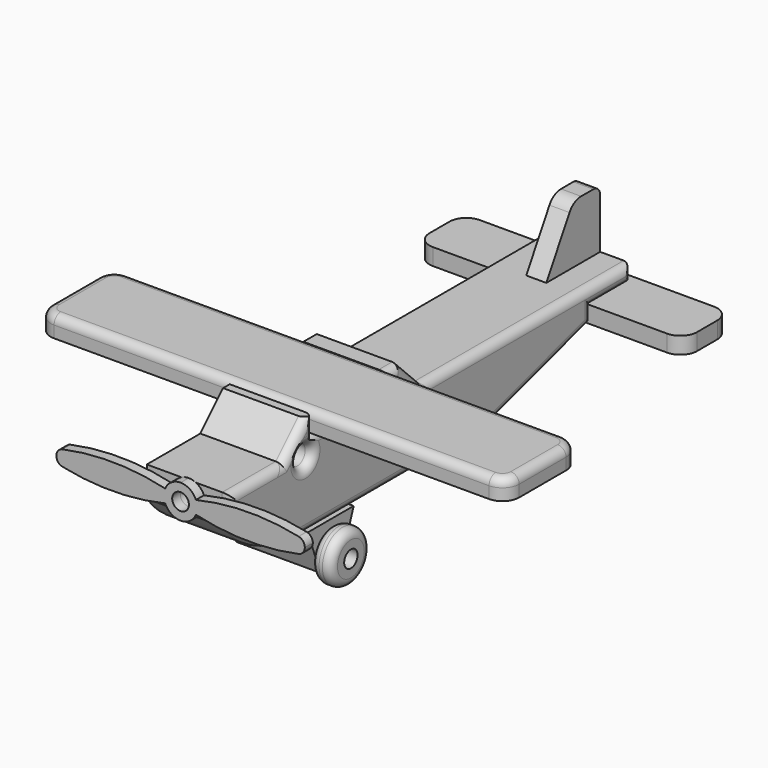
from build123d import *

# Parameters (mm, degrees)
F0_R           = 6
F1_DEPTH       = 25
F1_DEPTH_BACK  = 25
F2_W           = 55
F2_H           = 12
F3_DEPTH       = 140
F3_DEPTH_BACK  = 140
F4_R           = 10
F5_R           = 5
F6_W           = 35
F6_H           = 10
F7_DEPTH       = 80
F7_DEPTH_BACK  = 80
F8_R           = 10
F10_DEPTH      = 6
F10_DEPTH_BACK = 6
F11_R          = 10
F12_R          = 5
F13_R          = 5
F14_DEPTH      = 25
F14_DEPTH_BACK = 25
F15_R          = 15
F15_R_2        = 5
F16_DEPTH      = 12
F17_R          = 5
F18_R          = 5
F19_DEPTH      = 10
F20_R          = 5
F21_DEPTH      = 6
F22_R          = 4
F23_DEPTH      = 5
F24_R          = 4
F25_DEPTH      = 6
F26_T1_DEPTH   = 43.0048285071
F26_T3_DEPTH   = 162.520132507
F26_T5_DEPTH   = 117.2789705559
F26_T7_DEPTH   = 21.5024142536
F26_T9_DEPTH   = 42.5024142536
F26_T11_DEPTH  = 35.0048285071
F26_T13_DEPTH  = 35.0048285071
F26_T15_DEPTH  = 22.5024142536
F26_T17_DEPTH  = 55
F26_T20_ANGLE  = 66.2553378767
F26_T24_DEPTH  = 181.0048285071
F26_T29_DEPTH  = 49.0464590675
F26_T34_DEPTH  = 49.0464590675
F26_T39_DEPTH  = 65.0048285071
F26_T47_DEPTH  = 34.0048285071
F26_T52_DEPTH  = 42.5024142536
F26_T59_DEPTH  = 168.5024142536
F26_T63_DEPTH  = 49.0464590675
F26_T70_DEPTH  = 22.5024142536
F26_T74_DEPTH  = 67.5024142536
F26_T81_DEPTH  = 67.5024142536
F26_S83_R      = 6
F26_T84_DEPTH  = 35
F26_T87_DEPTH  = 22.5024142536
F26_S89_R      = 6
F26_T90_DEPTH  = 13
F26_T96_DEPTH  = 52.5024142536
F26_S98_R      = 6
F26_T99_DEPTH  = 28
F26_T102_DEPTH = 49.0464590675


# Not quite as in the source:
# - a fillet or chamfer that OpenCascade refuses, or shapes differently, is made with other operations: its cross-section is extruded or revolved along the edge and cut away or added


with BuildPart() as f1:
    # F0 (on Right) → F1 (new body, two sides)
    with BuildSketch(Plane.YZ) as f1_sk:
        with BuildLine():
            Line((-150, 18), (-150, 0))
            ThreePointArc((-150, 0), (-128.6521561512, -18.3853912602), (-101.266028276, -25))
            Line((-101.266028276, -25), (40, -25))
            Line((40, -25), (120, -1))
            Line((120, -1), (120, 8))
            Line((120, 8), (150, 8))
            Line((150, 8), (150, 18))
            Line((150, 18), (-6, 18))
            Line((-6, 18), (-23, 35))
            Line((-23, 35), (-33, 35))
            Line((-33, 35), (-33, 25))
            Line((-33, 25), (-88, 25))
            Line((-88, 25), (-88, 35))
            Line((-88, 35), (-93, 35))
            Line((-93, 35), (-110, 18))
            Line((-110, 18), (-150, 18))
        make_face()
        with Locations((-94, 15)):
            Circle(F0_R, mode=Mode.SUBTRACT)
    extrude(amount=F1_DEPTH)
    extrude(f1_sk.sketch, amount=-F1_DEPTH_BACK)

    # F18 (on face) → F19 (cut)
    with BuildSketch(Plane.XZ.offset(150)):
        with Locations((0, 9)):
            Circle(F18_R)
    extrude(amount=-F19_DEPTH, mode=Mode.SUBTRACT)

    # F24 (on face) → F25 (cut)
    with BuildSketch(Plane(origin=(0, 0, -25), x_dir=(1, 0, 0), z_dir=(0, 0, -1))):
        with Locations((-12, 75)):
            Circle(F24_R)
        with Locations((12, 75)):
            Circle(F24_R)
    extrude(amount=-F25_DEPTH, mode=Mode.SUBTRACT)

    # F26: fillet of radius 5 on 17 edges, made by hand

    # F26_s2 → F26_t1 (cut)
    with BuildSketch(Plane.XY.offset(-12.5024142536)):
        with BuildLine():
            ThreePointArc((19.9990343146, -150.0004), (23.5355339059, -148.5355339059), (25.0004, -144.9990343146))
            Line((25.0004, -144.9990343146), (25.5005365685, -144.9990343146))
            ThreePointArc((25.5005365685, -144.9990343146), (25.5001365685, -147.4995171573), (25.5001365685, -150))
            Line((25.5001365685, -150), (25, -150.5001365685))
            ThreePointArc((25, -150.5001365685), (22.4995171573, -150.5001365685), (19.9990343146, -150.5005365685))
            Line((19.9990343146, -150.5005365685), (19.9990343146, -150.0004))
        make_face()
    extrude(amount=F26_T1_DEPTH, mode=Mode.SUBTRACT)

    # F26_s4 → F26_t3 (cut)
    with BuildSketch(Plane.XZ.offset(-61.254104231)):
        with BuildLine():
            ThreePointArc((25.0004, -19.9990343146), (23.5355339059, -23.5355339059), (19.9990343146, -25.0004))
            Line((19.9990343146, -25.0004), (19.9990343146, -25.5005365685))
            ThreePointArc((19.9990343146, -25.5005365685), (22.4995171573, -25.5001365685), (25, -25.5001365685))
            Line((25, -25.5001365685), (25.5001365685, -25))
            ThreePointArc((25.5001365685, -25), (25.5001365685, -22.4995171573), (25.5005365685, -19.9990343146))
            Line((25.5005365685, -19.9990343146), (25.0004, -19.9990343146))
        make_face()
    extrude(amount=F26_T3_DEPTH, mode=Mode.SUBTRACT)

    # F26_s6 → F26_t5 (cut)
    with BuildSketch(Plane(origin=(0, 9.4587740601, 2.837632218), x_dir=(1, 0, 0), z_dir=(0, 0.9578262852, 0.2873478856))):
        with BuildLine():
            ThreePointArc((25.0004, 30.4386068678), (23.5355339059, 33.9751064591), (19.9990343146, 35.4399725532))
            Line((19.9990343146, 35.4399725532), (19.9990343146, 35.9401091217))
            ThreePointArc((19.9990343146, 35.9401091217), (22.4995171573, 35.9397091217), (25, 35.9397091217))
            Line((25, 35.9397091217), (25.5001365685, 35.4395725532))
            ThreePointArc((25.5001365685, 35.4395725532), (25.5001365685, 32.9390897105), (25.5005365685, 30.4386068678))
            Line((25.5005365685, 30.4386068678), (25.0004, 30.4386068678))
        make_face()
    extrude(amount=F26_T5_DEPTH, mode=Mode.SUBTRACT)

    # F26_s8 → F26_t7 (cut)
    with BuildSketch(Plane.XY.offset(-13.5024142536)):
        with BuildLine():
            ThreePointArc((25.0004, 114.9990343146), (23.5355339059, 118.5355339059), (19.9990343146, 120.0004))
            Line((19.9990343146, 120.0004), (19.9990343146, 120.5005365685))
            ThreePointArc((19.9990343146, 120.5005365685), (22.4995171573, 120.5001365685), (25, 120.5001365685))
            Line((25, 120.5001365685), (25.5001365685, 120))
            ThreePointArc((25.5001365685, 120), (25.5001365685, 117.4995171573), (25.5005365685, 114.9990343146))
            Line((25.5005365685, 114.9990343146), (25.0004, 114.9990343146))
        make_face()
    extrude(amount=F26_T7_DEPTH, mode=Mode.SUBTRACT)

    # F26_s10 → F26_t9 (cut)
    with BuildSketch(Plane.XZ.offset(-162.5024142536)):
        with BuildLine():
            ThreePointArc((25.0004, 13.0009656854), (23.5355339059, 9.4644660941), (19.9990343146, 7.9996))
            Line((19.9990343146, 7.9996), (19.9990343146, 7.4994634315))
            ThreePointArc((19.9990343146, 7.4994634315), (22.4995171573, 7.4998634315), (25, 7.4998634315))
            Line((25, 7.4998634315), (25.5001365685, 8))
            ThreePointArc((25.5001365685, 8), (25.5001365685, 10.5004828427), (25.5005365685, 13.0009656854))
            Line((25.5005365685, 13.0009656854), (25.0004, 13.0009656854))
        make_face()
    extrude(amount=F26_T9_DEPTH, mode=Mode.SUBTRACT)

    # F26_s12 → F26_t11 (cut)
    with BuildSketch(Plane.XY.offset(-4.5024142536)):
        with BuildLine():
            ThreePointArc((25.0004, 144.9990343146), (23.5355339059, 148.5355339059), (19.9990343146, 150.0004))
            Line((19.9990343146, 150.0004), (19.9990343146, 150.5005365685))
            ThreePointArc((19.9990343146, 150.5005365685), (22.4995171573, 150.5001365685), (25, 150.5001365685))
            Line((25, 150.5001365685), (25.5001365685, 150))
            ThreePointArc((25.5001365685, 150), (25.5001365685, 147.4995171573), (25.5005365685, 144.9990343146))
            Line((25.5005365685, 144.9990343146), (25.0004, 144.9990343146))
        make_face()
    extrude(amount=F26_T11_DEPTH, mode=Mode.SUBTRACT)

    # F26_s14 → F26_t13 (cut)
    with BuildSketch(Plane.XZ.offset(10.4975857464)):
        with BuildLine():
            ThreePointArc((25.0004, 29.9990343146), (23.5355339059, 33.5355339059), (19.9990343146, 35.0004))
            Line((19.9990343146, 35.0004), (19.9990343146, 35.5005365685))
            ThreePointArc((19.9990343146, 35.5005365685), (22.4995171573, 35.5001365685), (25, 35.5001365685))
            Line((25, 35.5001365685), (25.5001365685, 35))
            ThreePointArc((25.5001365685, 35), (25.5001365685, 32.4995171573), (25.5005365685, 29.9990343146))
            Line((25.5005365685, 29.9990343146), (25.0004, 29.9990343146))
        make_face()
    extrude(amount=F26_T13_DEPTH, mode=Mode.SUBTRACT)

    # F26_s16 → F26_t15 (cut)
    with BuildSketch(Plane.XY.offset(25)):
        with BuildLine():
            ThreePointArc((25.0004, -27.9990343146), (23.5355339059, -31.5355339059), (19.9990343146, -33.0004))
            Line((19.9990343146, -33.0004), (19.9990343146, -33.5005365685))
            ThreePointArc((19.9990343146, -33.5005365685), (22.4995171573, -33.5001365685), (25, -33.5001365685))
            Line((25, -33.5001365685), (25.5001365685, -33))
            ThreePointArc((25.5001365685, -33), (25.5001365685, -30.4995171573), (25.5005365685, -27.9990343146))
            Line((25.5005365685, -27.9990343146), (25.0004, -27.9990343146))
        make_face()
        with BuildLine():
            ThreePointArc((25.0004, -93.0009656854), (23.5355339059, -89.4644660941), (19.9990343146, -87.9996))
            Line((19.9990343146, -87.9996), (19.9990343146, -87.4994634315))
            ThreePointArc((19.9990343146, -87.4994634315), (22.4995171573, -87.4998634315), (25, -87.4998634315))
            Line((25, -87.4998634315), (25.5001365685, -88))
            ThreePointArc((25.5001365685, -88), (25.5001365685, -90.5004828427), (25.5005365685, -93.0009656854))
            Line((25.5005365685, -93.0009656854), (25.0004, -93.0009656854))
        make_face()
    extrude(amount=F26_T15_DEPTH, mode=Mode.SUBTRACT)

    # F26_s18 → F26_t17 (cut)
    with BuildSketch(Plane.XZ.offset(33)):
        with BuildLine():
            ThreePointArc((25.0004, 19.9990343146), (23.5355339059, 23.5355339059), (19.9990343146, 25.0004))
            Line((19.9990343146, 25.0004), (19.9990343146, 25.5005365685))
            ThreePointArc((19.9990343146, 25.5005365685), (22.4995171573, 25.5001365685), (25, 25.5001365685))
            Line((25, 25.5001365685), (25.5001365685, 25))
            ThreePointArc((25.5001365685, 25), (25.5001365685, 22.4995171573), (25.5005365685, 19.9990343146))
            Line((25.5005365685, 19.9990343146), (25.0004, 19.9990343146))
        make_face()
    extrude(amount=F26_T17_DEPTH, mode=Mode.SUBTRACT)

    # F26_s19 → F26_t20 (revolve, cut)
    with BuildSketch(Plane(origin=(0, -29.3190407601, 66.6494319351), x_dir=(1, 0, 0), z_dir=(0, -0.4026614145, 0.9153489964))):
        with BuildLine():
            ThreePointArc((25.0004, -133.5996421648), (23.5355339059, -137.1361417561), (19.9990343146, -138.6010078502))
            Line((19.9990343146, -138.6010078502), (19.9990343146, -139.1011444188))
            ThreePointArc((19.9990343146, -139.1011444188), (22.4995171573, -139.1007444188), (25, -139.1007444188))
            Line((25, -139.1007444188), (25.5001365685, -138.6006078502))
            ThreePointArc((25.5001365685, -138.6006078502), (25.5001365685, -136.1001250075), (25.5005365685, -133.5996421648))
            Line((25.5005365685, -133.5996421648), (25.0004, -133.5996421648))
        make_face()
    revolve(axis=Axis((25, -101.266028276, 35), (1, 0, 0)), revolution_arc=F26_T20_ANGLE, mode=Mode.SUBTRACT)


with BuildPart() as f3:
    # F2 (on Right) → F3 (new body, two sides)
    with BuildSketch(Plane.YZ) as f3_sk:
        with Locations((-60.5, 31)):
            Rectangle(F2_W, F2_H)
    extrude(amount=F3_DEPTH)
    extrude(f3_sk.sketch, amount=-F3_DEPTH_BACK)

    # F4
    f4_edges = [f3.edges().sort_by_distance(p)[0] for p in [
        (140, -88, 31),
        (140, -33, 31),
        (-140, -88, 31),
        (-140, -33, 31),
    ]]
    fillet(f4_edges, radius=F4_R)

    # F5
    f5_edges = [f3.edges().sort_by_distance(p)[0] for p in [
        (0, -33, 37),
        (137.071068, -35.928932, 37),
        (-137.071068, -35.928932, 37),
        (140, -60.5, 37),
        (-140, -60.5, 37),
        (137.071068, -85.071068, 37),
        (-137.071068, -85.071068, 37),
        (0, -88, 37),
    ]]
    fillet(f5_edges, radius=F5_R)


with BuildPart() as f7:
    # F6 (on Right) → F7 (new body, two sides)
    with BuildSketch(Plane.YZ) as f7_sk:
        with Locations((137.5, 3)):
            Rectangle(F6_W, F6_H)
    extrude(amount=F7_DEPTH)
    extrude(f7_sk.sketch, amount=-F7_DEPTH_BACK)

    # F8
    f8_edges = [f7.edges().sort_by_distance(p)[0] for p in [
        (80, 120, 3),
        (80, 155, 3),
        (-80, 155, 3),
        (-80, 120, 3),
    ]]
    fillet(f8_edges, radius=F8_R)


with BuildPart() as f10:
    # F9 (on Right) → F10 (new body, two sides)
    with BuildSketch(Plane.YZ) as f10_sk:
        Polygon((130, 53), (109.7927405784, 18), (150, 18), (150, 53), align=None)
    extrude(amount=F10_DEPTH)
    extrude(f10_sk.sketch, amount=-F10_DEPTH_BACK)

    # F11
    f11_edges = [f10.edges().sort_by_distance(p)[0] for p in [
        (0, 130, 53),
    ]]
    fillet(f11_edges, radius=F11_R)

    # F12
    f12_edges = [f10.edges().sort_by_distance(p)[0] for p in [
        (0, 150, 53),
    ]]
    fillet(f12_edges, radius=F12_R)


with BuildPart() as f14:
    # F13 (on Right) → F14 (new body, two sides)
    with BuildSketch(Plane.YZ) as f14_sk:
        Polygon((-67, -50), (-57.9007441433, -25), (-92.0992558567, -25), (-83, -50), align=None)
        with Locations((-75, -42)):
            Circle(F13_R, mode=Mode.SUBTRACT)
    extrude(amount=F14_DEPTH)
    extrude(f14_sk.sketch, amount=-F14_DEPTH_BACK)

    # F22 (on face) → F23 (cut)
    with BuildSketch(Plane.XY.offset(-25)):
        with Locations((-12, -75)):
            Circle(F22_R)
        with Locations((12, -75)):
            Circle(F22_R)
    extrude(amount=-F23_DEPTH, mode=Mode.SUBTRACT)


with BuildPart() as f16:
    # F15 (on face) → F16 (new body)
    with BuildSketch(Plane.YZ.offset(25)):
        with Locations((-75, -42)):
            Circle(F15_R)
        with Locations((-75, -42)):
            Circle(F15_R_2, mode=Mode.SUBTRACT)
    extrude(amount=F16_DEPTH)

    # F17
    f17_edges = [f16.edges().sort_by_distance(p)[0] for p in [
        (31, -60, -42),
        (25, -90, -42),
        (37, -90, -42),
    ]]
    fillet(f17_edges, radius=F17_R)


with BuildPart() as f21:
    # F20 (on face) → F21 (new body)
    with BuildSketch(Plane.XZ.offset(150)):
        with BuildLine():
            ThreePointArc((70.5365811846, 13.605655082), (39.8328024938, 16.6540772066), (9.2069454802, 12.9028393414))
            ThreePointArc((9.2069454802, 12.9028393414), (5.5213950495, 17.3375174187), (0, 19))
            ThreePointArc((0, 19), (-5.5213950495, 17.3375174187), (-9.2069454802, 12.9028393414))
            ThreePointArc((-9.2069454802, 12.9028393414), (-39.8328024938, 16.6540772066), (-70.5365811846, 13.605655082))
            ThreePointArc((-70.5365811846, 13.605655082), (-73.2169993023, 11.9632563595), (-74.2663927448, 9))
            ThreePointArc((-74.2663927448, 9), (-73.2169993023, 6.0367436405), (-70.5365811846, 4.394344918))
            ThreePointArc((-70.5365811846, 4.394344918), (-39.8328024938, 1.3459227934), (-9.2069454802, 5.0971606586))
            ThreePointArc((-9.2069454802, 5.0971606586), (-5.5213950495, 0.6624825813), (0, -1))
            ThreePointArc((0, -1), (5.5213950495, 0.6624825813), (9.2069454802, 5.0971606586))
            ThreePointArc((9.2069454802, 5.0971606586), (39.8328024938, 1.3459227934), (70.5365811846, 4.394344918))
            ThreePointArc((70.5365811846, 4.394344918), (73.2169993023, 6.0367436405), (74.2663927448, 9))
            ThreePointArc((74.2663927448, 9), (73.2169993023, 11.9632563595), (70.5365811846, 13.605655082))
        make_face()
        with Locations((0, 9)):
            Circle(F20_R, mode=Mode.SUBTRACT)
    extrude(amount=F21_DEPTH)


with BuildPart() as f26_tool22:
    # F26_s23 → F26_t24 (new body)
    with BuildSketch(Plane.XZ.offset(-162.5024142536)):
        with BuildLine():
            ThreePointArc((25.0004, 12.9990343146), (23.5355339059, 16.5355339059), (19.9990343146, 18.0004))
            Line((19.9990343146, 18.0004), (19.9990343146, 18.5005365685))
            ThreePointArc((19.9990343146, 18.5005365685), (22.4995171573, 18.5001365685), (25, 18.5001365685))
            Line((25, 18.5001365685), (25.5001365685, 18))
            ThreePointArc((25.5001365685, 18), (25.5001365685, 15.4995171573), (25.5005365685, 12.9990343146))
            Line((25.5005365685, 12.9990343146), (25.0004, 12.9990343146))
        make_face()
    extrude(amount=F26_T24_DEPTH)

    split(bisect_by=Plane(origin=(0, 6, 6), x_dir=(1, 0, 0), z_dir=(0, 0.7071067812, 0.7071067812)), keep=Keep.TOP)


with BuildPart() as f1_1:
    add(f1.part)

    # F26_t21: cut F26_tool22
    add(f26_tool22.part, mode=Mode.SUBTRACT)


with BuildPart() as f26_tool27:
    # F26_s28 → F26_t29 (new body)
    with BuildSketch(Plane(origin=(0, -3.1594581001, 3.1594581001), x_dir=(1, 0, 0), z_dir=(0, -0.7071067812, 0.7071067812))):
        with BuildLine():
            ThreePointArc((25.0004, 3.4843156888), (23.5355339059, 7.0208152802), (19.9990343146, 8.4856813742))
            Line((19.9990343146, 8.4856813742), (19.9990343146, 8.9858179428))
            ThreePointArc((19.9990343146, 8.9858179428), (22.4995171573, 8.9854179428), (25, 8.9854179428))
            Line((25, 8.9854179428), (25.5001365685, 8.4852813742))
            ThreePointArc((25.5001365685, 8.4852813742), (25.5001365685, 5.9847985315), (25.5005365685, 3.4843156888))
            Line((25.5005365685, 3.4843156888), (25.0004, 3.4843156888))
        make_face()
    extrude(amount=F26_T29_DEPTH)

    split(bisect_by=Plane.XY.offset(18), keep=Keep.TOP)


with BuildPart() as f1_2:
    add(f1_1.part)

    # F26_t26: cut F26_tool27
    add(f26_tool27.part, mode=Mode.SUBTRACT)


with BuildPart() as f26_tool32:
    # F26_s33 → F26_t34 (new body)
    with BuildSketch(Plane(origin=(0, -20.1594581001, -20.1594581001), x_dir=(1, 0, 0), z_dir=(0, -0.7071067812, -0.7071067812))):
        with BuildLine():
            ThreePointArc((25.0004, 85.5087023065), (23.5355339059, 89.0452018978), (19.9990343146, 90.5100679919))
            Line((19.9990343146, 90.5100679919), (19.9990343146, 91.0102045604))
            ThreePointArc((19.9990343146, 91.0102045604), (22.4995171573, 91.0098045604), (25, 91.0098045604))
            Line((25, 91.0098045604), (25.5001365685, 90.5096679919))
            ThreePointArc((25.5001365685, 90.5096679919), (25.5001365685, 88.0091851492), (25.5005365685, 85.5087023065))
            Line((25.5005365685, 85.5087023065), (25.0004, 85.5087023065))
        make_face()
    extrude(amount=F26_T34_DEPTH)

    split(bisect_by=Plane.XY.offset(18), keep=Keep.TOP)


with BuildPart() as f1_3:
    add(f1_2.part)

    # F26_t31: cut F26_tool32
    add(f26_tool32.part, mode=Mode.SUBTRACT)


with BuildPart() as f26_tool37:
    # F26_s38 → F26_t39 (new body)
    with BuildSketch(Plane.XZ.offset(97.4975857464)):
        with BuildLine():
            ThreePointArc((19.9990343146, 18.0004), (23.5355339059, 16.5355339059), (25.0004, 12.9990343146))
            Line((25.0004, 12.9990343146), (25.5005365685, 12.9990343146))
            ThreePointArc((25.5005365685, 12.9990343146), (25.5001365685, 15.4995171573), (25.5001365685, 18))
            Line((25.5001365685, 18), (25, 18.5001365685))
            ThreePointArc((25, 18.5001365685), (22.4995171573, 18.5001365685), (19.9990343146, 18.5005365685))
            Line((19.9990343146, 18.5005365685), (19.9990343146, 18.0004))
        make_face()
    extrude(amount=F26_T39_DEPTH)

    split(bisect_by=Plane(origin=(0, -64, 64), x_dir=(1, 0, 0), z_dir=(0, -0.7071067812, 0.7071067812)), keep=Keep.TOP)


with BuildPart() as f1_4:
    add(f1_3.part)

    # F26_t36: cut F26_tool37
    add(f26_tool37.part, mode=Mode.SUBTRACT)

    # F26_s41 → F26_t42 (revolve, cut)
    with BuildSketch(Plane.XY.offset(15)):
        with BuildLine():
            ThreePointArc((25.0004, -82.9990343146), (23.5355339059, -86.5355339059), (19.9990343146, -88.0004))
            Line((19.9990343146, -88.0004), (19.9990343146, -88.5005365685))
            ThreePointArc((19.9990343146, -88.5005365685), (22.4995171573, -88.5001365685), (25, -88.5001365685))
            Line((25, -88.5001365685), (25.5001365685, -88))
            ThreePointArc((25.5001365685, -88), (25.5001365685, -85.4995171573), (25.5005365685, -82.9990343146))
            Line((25.5005365685, -82.9990343146), (25.0004, -82.9990343146))
        make_face()
    revolve(axis=Axis((25, -94, 15), (1, 0, 0)), mode=Mode.SUBTRACT)


with BuildPart() as f26_tool45:
    # F26_s46 → F26_t47 (new body)
    with BuildSketch(Plane.XY.offset(-13.5024142536)):
        with BuildLine():
            ThreePointArc((25.0004, 114.9990343146), (23.5355339059, 118.5355339059), (19.9990343146, 120.0004))
            Line((19.9990343146, 120.0004), (19.9990343146, 120.5005365685))
            ThreePointArc((19.9990343146, 120.5005365685), (22.4995171573, 120.5001365685), (25, 120.5001365685))
            Line((25, 120.5001365685), (25.5001365685, 120))
            ThreePointArc((25.5001365685, 120), (25.5001365685, 117.4995171573), (25.5005365685, 114.9990343146))
            Line((25.5005365685, 114.9990343146), (25.0004, 114.9990343146))
        make_face()
    extrude(amount=F26_T47_DEPTH)

    split(bisect_by=Plane.XY.offset(8), keep=Keep.TOP)

    split(bisect_by=Plane.XY.offset(18), keep=Keep.BOTTOM)


with BuildPart() as f26_tool50:
    # F26_s51 → F26_t52 (new body)
    with BuildSketch(Plane.XZ.offset(-107.4975857464)):
        with BuildLine():
            ThreePointArc((25.0004, 13.0009656854), (23.5355339059, 9.4644660941), (19.9990343146, 7.9996))
            Line((19.9990343146, 7.9996), (19.9990343146, 7.4994634315))
            ThreePointArc((19.9990343146, 7.4994634315), (22.4995171573, 7.4998634315), (25, 7.4998634315))
            Line((25, 7.4998634315), (25.5001365685, 8))
            ThreePointArc((25.5001365685, 8), (25.5001365685, 10.5004828427), (25.5005365685, 13.0009656854))
            Line((25.5005365685, 13.0009656854), (25.0004, 13.0009656854))
        make_face()
    extrude(amount=-F26_T52_DEPTH)

    split(bisect_by=Plane.XZ.offset(-120), keep=Keep.TOP)


with BuildPart() as f26_tool45_1:
    add(f26_tool45.part)

    # F26_t54: intersect F26_tool50
    add(f26_tool50.part, mode=Mode.INTERSECT)


with BuildPart() as f1_5:
    add(f1_4.part)

    # F26_t43: cut F26_tool45
    add(f26_tool45_1.part, mode=Mode.SUBTRACT)


with BuildPart() as f26_tool57:
    # F26_s58 → F26_t59 (new body)
    with BuildSketch(Plane.XZ.offset(-150)):
        with BuildLine():
            ThreePointArc((25.0004, 12.9990343146), (23.5355339059, 16.5355339059), (19.9990343146, 18.0004))
            Line((19.9990343146, 18.0004), (19.9990343146, 18.5005365685))
            ThreePointArc((19.9990343146, 18.5005365685), (22.4995171573, 18.5001365685), (25, 18.5001365685))
            Line((25, 18.5001365685), (25.5001365685, 18))
            ThreePointArc((25.5001365685, 18), (25.5001365685, 15.4995171573), (25.5005365685, 12.9990343146))
            Line((25.5005365685, 12.9990343146), (25.0004, 12.9990343146))
        make_face()
    extrude(amount=F26_T59_DEPTH)

    split(bisect_by=Plane(origin=(0, 6, 6), x_dir=(1, 0, 0), z_dir=(0, -0.7071067812, -0.7071067812)), keep=Keep.TOP)


with BuildPart() as f26_tool61:
    # F26_s62 → F26_t63 (new body)
    with BuildSketch(Plane(origin=(0, -3.1594581001, 3.1594581001), x_dir=(1, 0, 0), z_dir=(0, -0.7071067812, 0.7071067812))):
        with BuildLine():
            ThreePointArc((25.0004, 3.4843156888), (23.5355339059, 7.0208152802), (19.9990343146, 8.4856813742))
            Line((19.9990343146, 8.4856813742), (19.9990343146, 8.9858179428))
            ThreePointArc((19.9990343146, 8.9858179428), (22.4995171573, 8.9854179428), (25, 8.9854179428))
            Line((25, 8.9854179428), (25.5001365685, 8.4852813742))
            ThreePointArc((25.5001365685, 8.4852813742), (25.5001365685, 5.9847985315), (25.5005365685, 3.4843156888))
            Line((25.5005365685, 3.4843156888), (25.0004, 3.4843156888))
        make_face()
    extrude(amount=F26_T63_DEPTH)

    split(bisect_by=Plane.XY.offset(18), keep=Keep.BOTTOM)


with BuildPart() as f26_tool57_1:
    add(f26_tool57.part)

    # F26_t65: intersect F26_tool61
    add(f26_tool61.part, mode=Mode.INTERSECT)


with BuildPart() as f1_6:
    add(f1_5.part)

    # F26_t55: cut F26_tool57
    add(f26_tool57_1.part, mode=Mode.SUBTRACT)


with BuildPart() as f26_tool68:
    # F26_s69 → F26_t70 (new body)
    with BuildSketch(Plane.XY.offset(35)):
        with BuildLine():
            ThreePointArc((25.0004, -27.9990343146), (23.5355339059, -31.5355339059), (19.9990343146, -33.0004))
            Line((19.9990343146, -33.0004), (19.9990343146, -33.5005365685))
            ThreePointArc((19.9990343146, -33.5005365685), (22.4995171573, -33.5001365685), (25, -33.5001365685))
            Line((25, -33.5001365685), (25.5001365685, -33))
            ThreePointArc((25.5001365685, -33), (25.5001365685, -30.4995171573), (25.5005365685, -27.9990343146))
            Line((25.5005365685, -27.9990343146), (25.0004, -27.9990343146))
        make_face()
    extrude(amount=-F26_T70_DEPTH)

    split(bisect_by=Plane.XY.offset(25), keep=Keep.BOTTOM)


with BuildPart() as f26_tool72:
    # F26_s73 → F26_t74 (new body)
    with BuildSketch(Plane.XZ.offset(20.4975857464)):
        with BuildLine():
            ThreePointArc((25.0004, 19.9990343146), (23.5355339059, 23.5355339059), (19.9990343146, 25.0004))
            Line((19.9990343146, 25.0004), (19.9990343146, 25.5005365685))
            ThreePointArc((19.9990343146, 25.5005365685), (22.4995171573, 25.5001365685), (25, 25.5001365685))
            Line((25, 25.5001365685), (25.5001365685, 25))
            ThreePointArc((25.5001365685, 25), (25.5001365685, 22.4995171573), (25.5005365685, 19.9990343146))
            Line((25.5005365685, 19.9990343146), (25.0004, 19.9990343146))
        make_face()
    extrude(amount=F26_T74_DEPTH)

    split(bisect_by=Plane.XZ.offset(33), keep=Keep.BOTTOM)


with BuildPart() as f26_tool68_1:
    add(f26_tool68.part)

    # F26_t76: intersect F26_tool72
    add(f26_tool72.part, mode=Mode.INTERSECT)


with BuildPart() as f1_7:
    add(f1_6.part)

    # F26_t66: cut F26_tool68
    add(f26_tool68_1.part, mode=Mode.SUBTRACT)


with BuildPart() as f26_tool79:
    # F26_s80 → F26_t81 (new body)
    with BuildSketch(Plane.XZ.offset(33)):
        with BuildLine():
            ThreePointArc((25.0004, 19.9990343146), (23.5355339059, 23.5355339059), (19.9990343146, 25.0004))
            Line((19.9990343146, 25.0004), (19.9990343146, 25.5005365685))
            ThreePointArc((19.9990343146, 25.5005365685), (22.4995171573, 25.5001365685), (25, 25.5001365685))
            Line((25, 25.5001365685), (25.5001365685, 25))
            ThreePointArc((25.5001365685, 25), (25.5001365685, 22.4995171573), (25.5005365685, 19.9990343146))
            Line((25.5005365685, 19.9990343146), (25.0004, 19.9990343146))
        make_face()
    extrude(amount=F26_T81_DEPTH)

    split(bisect_by=Plane.XZ.offset(88), keep=Keep.TOP)

    # F26_s83 → F26_t84 (cut, symmetric)
    with BuildSketch(Plane.YZ.offset(22.7)):
        with Locations((-94, 15)):
            Circle(F26_S83_R)
    extrude(amount=F26_T84_DEPTH, both=True, mode=Mode.SUBTRACT)


with BuildPart() as f26_tool85:
    # F26_s86 → F26_t87 (new body)
    with BuildSketch(Plane.XY.offset(12.4975857464)):
        with BuildLine():
            ThreePointArc((25.0004, -93.0009656854), (23.5355339059, -89.4644660941), (19.9990343146, -87.9996))
            Line((19.9990343146, -87.9996), (19.9990343146, -87.4994634315))
            ThreePointArc((19.9990343146, -87.4994634315), (22.4995171573, -87.4998634315), (25, -87.4998634315))
            Line((25, -87.4998634315), (25.5001365685, -88))
            ThreePointArc((25.5001365685, -88), (25.5001365685, -90.5004828427), (25.5005365685, -93.0009656854))
            Line((25.5005365685, -93.0009656854), (25.0004, -93.0009656854))
        make_face()
    extrude(amount=F26_T87_DEPTH)

    split(bisect_by=Plane.XY.offset(25), keep=Keep.BOTTOM)

    # F26_s89 → F26_t90 (cut, symmetric)
    with BuildSketch(Plane.YZ.offset(22.7)):
        with Locations((-94, 15)):
            Circle(F26_S89_R)
    extrude(amount=F26_T90_DEPTH, both=True, mode=Mode.SUBTRACT)


with BuildPart() as f26_tool79_1:
    add(f26_tool79.part)

    # F26_t91: intersect F26_tool85
    add(f26_tool85.part, mode=Mode.INTERSECT)


with BuildPart() as f1_8:
    add(f1_7.part)

    # F26_t77: cut F26_tool79
    add(f26_tool79_1.part, mode=Mode.SUBTRACT)


with BuildPart() as f26_tool94:
    # F26_s95 → F26_t96 (new body)
    with BuildSketch(Plane.XZ.offset(97.4975857464)):
        with BuildLine():
            ThreePointArc((19.9990343146, 18.0004), (23.5355339059, 16.5355339059), (25.0004, 12.9990343146))
            Line((25.0004, 12.9990343146), (25.5005365685, 12.9990343146))
            ThreePointArc((25.5005365685, 12.9990343146), (25.5001365685, 15.4995171573), (25.5001365685, 18))
            Line((25.5001365685, 18), (25, 18.5001365685))
            ThreePointArc((25, 18.5001365685), (22.4995171573, 18.5001365685), (19.9990343146, 18.5005365685))
            Line((19.9990343146, 18.5005365685), (19.9990343146, 18.0004))
        make_face()
    extrude(amount=F26_T96_DEPTH)

    split(bisect_by=Plane(origin=(0, -64, 64), x_dir=(1, 0, 0), z_dir=(0, 0.7071067812, -0.7071067812)), keep=Keep.TOP)

    # F26_s98 → F26_t99 (cut, symmetric)
    with BuildSketch(Plane.YZ.offset(22.7)):
        with Locations((-94, 15)):
            Circle(F26_S98_R)
    extrude(amount=F26_T99_DEPTH, both=True, mode=Mode.SUBTRACT)


with BuildPart() as f26_tool100:
    # F26_s101 → F26_t102 (new body)
    with BuildSketch(Plane(origin=(0, -20.1594581001, -20.1594581001), x_dir=(1, 0, 0), z_dir=(0, -0.7071067812, -0.7071067812))):
        with BuildLine():
            ThreePointArc((25.0004, 85.5087023065), (23.5355339059, 89.0452018978), (19.9990343146, 90.5100679919))
            Line((19.9990343146, 90.5100679919), (19.9990343146, 91.0102045604))
            ThreePointArc((19.9990343146, 91.0102045604), (22.4995171573, 91.0098045604), (25, 91.0098045604))
            Line((25, 91.0098045604), (25.5001365685, 90.5096679919))
            ThreePointArc((25.5001365685, 90.5096679919), (25.5001365685, 88.0091851492), (25.5005365685, 85.5087023065))
            Line((25.5005365685, 85.5087023065), (25.0004, 85.5087023065))
        make_face()
    extrude(amount=F26_T102_DEPTH)

    split(bisect_by=Plane.XY.offset(18), keep=Keep.BOTTOM)


with BuildPart() as f26_tool94_1:
    add(f26_tool94.part)

    # F26_t104: intersect F26_tool100
    add(f26_tool100.part, mode=Mode.INTERSECT)


with BuildPart() as f1_9:
    add(f1_8.part)

    # F26_t92: cut F26_tool94
    add(f26_tool94_1.part, mode=Mode.SUBTRACT)


solid = Compound([f3.part, f7.part, f10.part, f14.part, f16.part, f21.part, f1_9.part])
